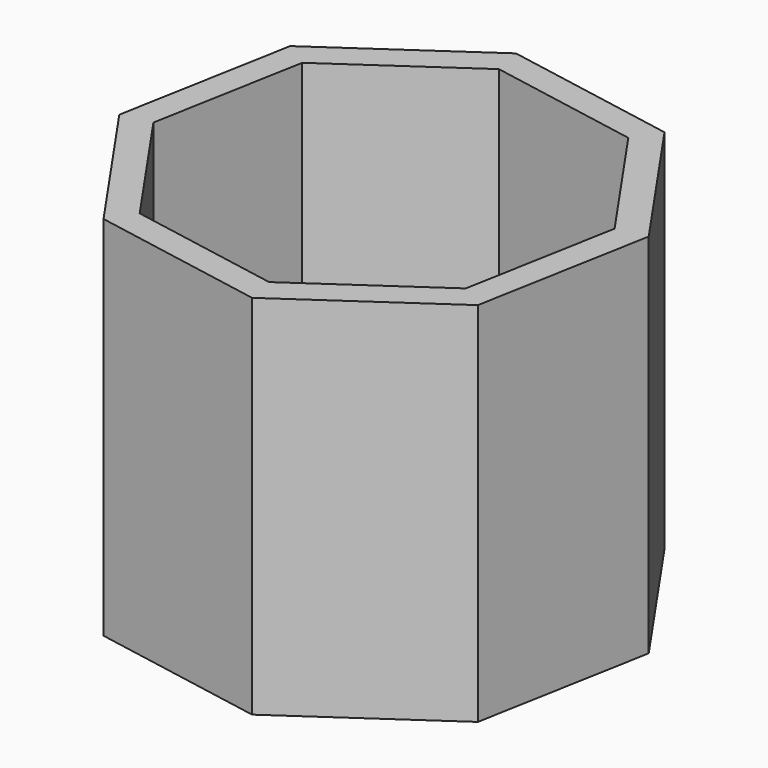
from build123d import *

# Parameters (mm, degrees)
F1_DEPTH = 127
F2_T     = -9.525


# Not quite as in the source:
# - a length typed as a fraction of an inch, garbled in the dataset ("3 / 203.2 mm" for 3/8 in), is restored


with BuildPart() as f1:
    # F0 (on Top) → F1 (new body)
    with BuildSketch(Plane.XY):
        Polygon((-25.8614264401, 39.6310188183), (-60.6637008516, 89.9540535799), (-120.8563842186, 100.9288884727), (-171.1794189802, 66.1266140612), (-182.154253873, 5.9339306942), (-147.3519794615, -44.3891040675), (-87.1592960945, -55.3639389602), (-36.8362613329, -20.5616645487), align=None)
    extrude(amount=F1_DEPTH)

    # F2
    f2_openings = [f1.faces().sort_by_distance(p)[0] for p in [
        (-104.00784, 22.782475, 127),
    ]]
    offset(amount=F2_T, openings=f2_openings)


solid = f1.part
